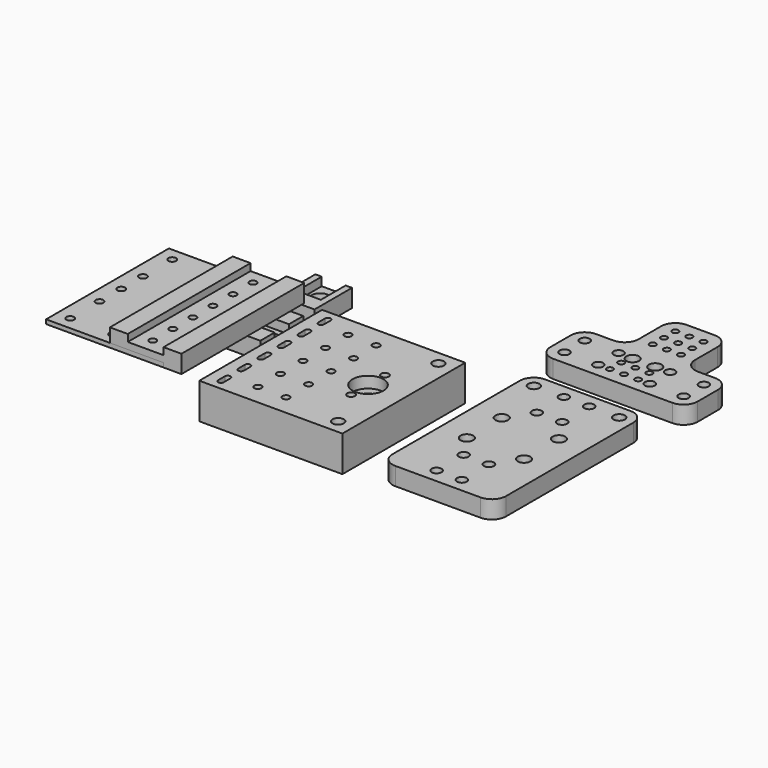
from build123d import *

# Parameters (mm, degrees)
F1_R      = 2.5
F2_DEPTH  = 12.7
F3_W      = 25.4
F3_H      = 109
F3_R      = 2.5
F4_DEPTH  = 5
F0_R      = 2.55
F0_R_2    = 4
F0_R_3    = 2.75
F0_R_4    = 11
F0_R_5    = 5.2625
F5_DEPTH  = 25.4
F6_DEPTH  = 8
F7_R      = 2.75
F8_DEPTH  = 3
F9_R      = 3.5
F9_R_2    = 4.5
F9_R_3    = 4
F9_R_4    = 2.25
F9_R_5    = 2.75
F10_DEPTH = 12.7
F11_DEPTH = 5
F12_R     = 3.5
F12_R_2   = 2.25
F12_R_3   = 4.5
F12_R_4   = 2.5
F12_R_5   = 2
F13_DEPTH = 12.7
F14_DEPTH = 5
F15_W     = 26
F15_H     = 12.7
F15_R     = 2.25
F16_DEPTH = 12.7
F17_DEPTH = 6.35
F18_W     = 17
F18_H     = 22
F18_R     = 6.25
F19_DEPTH = 12.7
F20_DEPTH = 6


# Not quite as in the source:
# - a length typed as a fraction of an inch, garbled in the dataset ("3 / 203.2 mm" for 3/8 in), is restored


with BuildPart() as f2:
    # F1 (on Top) → F2 (new body)
    with BuildSketch(Plane.XY):
        Polygon((-50.8, 0), (-25.4, 0), (-12.7, 0), (-12.7, 109), (-25.4, 109), (-50.8, 109), (-63.5, 109), (-63.5, 0), align=None)
        with Locations((-41.06, 10)):
            Circle(F1_R, mode=Mode.SUBTRACT)
        with Locations((-41.06, 27.8)):
            Circle(F1_R, mode=Mode.SUBTRACT)
        with Locations((-41.06, 45.6)):
            Circle(F1_R, mode=Mode.SUBTRACT)
        with Locations((-41.06, 63.4)):
            Circle(F1_R, mode=Mode.SUBTRACT)
        with Locations((-41.06, 81.2)):
            Circle(F1_R, mode=Mode.SUBTRACT)
        with Locations((-41.06, 99)):
            Circle(F1_R, mode=Mode.SUBTRACT)
    extrude(amount=F2_DEPTH)

    # F3 (on face) → F4 (cut)
    with BuildSketch(Plane.XY.offset(12.7)):
        with Locations((-38.1, 54.5)):
            Rectangle(F3_W, F3_H)
        with Locations((-41.06, 10)):
            Circle(F3_R, mode=Mode.SUBTRACT)
        with Locations((-41.06, 27.8)):
            Circle(F3_R, mode=Mode.SUBTRACT)
        with Locations((-41.06, 45.6)):
            Circle(F3_R, mode=Mode.SUBTRACT)
        with Locations((-41.06, 63.4)):
            Circle(F3_R, mode=Mode.SUBTRACT)
        with Locations((-41.06, 81.2)):
            Circle(F3_R, mode=Mode.SUBTRACT)
        with Locations((-41.06, 99)):
            Circle(F3_R, mode=Mode.SUBTRACT)
    extrude(amount=-F4_DEPTH, mode=Mode.SUBTRACT)


with BuildPart() as f5:
    # F0 (on Top) → F5 (new body)
    with BuildSketch(Plane.XY):
        Polygon((0, 109), (0, 0), (101.6, 0), (101.6, 102.8568819165), (101.6, 109), align=None)
        with BuildLine():
            ThreePointArc((7.74, 13), (9.74, 15), (11.74, 13))
            Line((11.74, 13), (11.74, 7))
            ThreePointArc((11.74, 7), (9.74, 5), (7.74, 7))
            Line((7.74, 7), (7.74, 13))
        make_face(mode=Mode.SUBTRACT)
        with Locations((30, 14.5)):
            Circle(F0_R, mode=Mode.SUBTRACT)
        with Locations((50, 14.5)):
            Circle(F0_R, mode=Mode.SUBTRACT)
        with BuildLine():
            ThreePointArc((7.74, 30.8), (9.74, 32.8), (11.74, 30.8))
            Line((11.74, 30.8), (11.74, 24.8))
            ThreePointArc((11.74, 24.8), (9.74, 22.8), (7.74, 24.8))
            Line((7.74, 24.8), (7.74, 30.8))
        make_face(mode=Mode.SUBTRACT)
        with BuildLine():
            ThreePointArc((7.74, 48.6), (9.74, 50.6), (11.74, 48.6))
            Line((11.74, 48.6), (11.74, 42.6))
            ThreePointArc((11.74, 42.6), (9.74, 40.6), (7.74, 42.6))
            Line((7.74, 42.6), (7.74, 48.6))
        make_face(mode=Mode.SUBTRACT)
        with Locations((30, 34.5)):
            Circle(F0_R, mode=Mode.SUBTRACT)
        with Locations((50, 34.5)):
            Circle(F0_R, mode=Mode.SUBTRACT)
        with Locations((90.6, 10)):
            Circle(F0_R_2, mode=Mode.SUBTRACT)
        with Locations((76.2, 39.5)):
            Circle(F0_R_3, mode=Mode.SUBTRACT)
        with BuildLine():
            ThreePointArc((7.74, 66.4), (9.74, 68.4), (11.74, 66.4))
            Line((11.74, 66.4), (11.74, 60.4))
            ThreePointArc((11.74, 60.4), (9.74, 58.4), (7.74, 60.4))
            Line((7.74, 60.4), (7.74, 66.4))
        make_face(mode=Mode.SUBTRACT)
        with BuildLine():
            ThreePointArc((7.74, 84.2), (9.74, 86.2), (11.74, 84.2))
            Line((11.74, 84.2), (11.74, 78.2))
            ThreePointArc((11.74, 78.2), (9.74, 76.2), (7.74, 78.2))
            Line((7.74, 78.2), (7.74, 84.2))
        make_face(mode=Mode.SUBTRACT)
        with Locations((30, 54.5)):
            Circle(F0_R, mode=Mode.SUBTRACT)
        with Locations((50, 54.5)):
            Circle(F0_R, mode=Mode.SUBTRACT)
        with Locations((30, 74.5)):
            Circle(F0_R, mode=Mode.SUBTRACT)
        with Locations((50, 74.5)):
            Circle(F0_R, mode=Mode.SUBTRACT)
        with BuildLine():
            ThreePointArc((7.74, 102), (9.74, 104), (11.74, 102))
            Line((11.74, 102), (11.74, 96))
            ThreePointArc((11.74, 96), (9.74, 94), (7.74, 96))
            Line((7.74, 96), (7.74, 102))
        make_face(mode=Mode.SUBTRACT)
        with Locations((30, 94.5)):
            Circle(F0_R, mode=Mode.SUBTRACT)
        with Locations((50, 94.5)):
            Circle(F0_R, mode=Mode.SUBTRACT)
        with Locations((76.2, 54.5)):
            Circle(F0_R_4, mode=Mode.SUBTRACT)
        with Locations((76.2, 69.5)):
            Circle(F0_R_3, mode=Mode.SUBTRACT)
        with Locations((90.6, 99)):
            Circle(F0_R_2, mode=Mode.SUBTRACT)
        with Locations((76.2, 54.5)):
            Circle(F0_R_4)
        with Locations((76.2, 54.5)):
            Circle(F0_R_5, mode=Mode.SUBTRACT)
    extrude(amount=-F5_DEPTH)

    # F0 (on Top) → F6 (cut)
    with BuildSketch(Plane.XY):
        with Locations((76.2, 54.5)):
            Circle(F0_R_4)
        with Locations((76.2, 54.5)):
            Circle(F0_R_5, mode=Mode.SUBTRACT)
    extrude(amount=-F6_DEPTH, mode=Mode.SUBTRACT)


with BuildPart() as f8:
    # F7 (on face) → F8 (new body)
    with BuildSketch(Plane.XY):
        Polygon((-25.4, 0), (-25.4, 109), (-58.8, 109), (-83.8, 109), (-108.8, 109), (-108.8, 0), align=None)
        with Locations((-99.05, 9.25)):
            Circle(F7_R, mode=Mode.SUBTRACT)
        with Locations((-68.55, 9.25)):
            Circle(F7_R, mode=Mode.SUBTRACT)
        with Locations((-35.14, 10)):
            Circle(F7_R, mode=Mode.SUBTRACT)
        with Locations((-99.05, 35.25)):
            Circle(F7_R, mode=Mode.SUBTRACT)
        with Locations((-68.55, 35.25)):
            Circle(F7_R, mode=Mode.SUBTRACT)
        with Locations((-35.14, 27.8)):
            Circle(F7_R, mode=Mode.SUBTRACT)
        with Locations((-35.14, 45.6)):
            Circle(F7_R, mode=Mode.SUBTRACT)
        with Locations((-99.05, 54.5)):
            Circle(F7_R, mode=Mode.SUBTRACT)
        with Locations((-68.55, 54.5)):
            Circle(F7_R, mode=Mode.SUBTRACT)
        with Locations((-99.05, 73.75)):
            Circle(F7_R, mode=Mode.SUBTRACT)
        with Locations((-68.55, 73.75)):
            Circle(F7_R, mode=Mode.SUBTRACT)
        with Locations((-35.14, 63.4)):
            Circle(F7_R, mode=Mode.SUBTRACT)
        with Locations((-35.14, 81.2)):
            Circle(F7_R, mode=Mode.SUBTRACT)
        with Locations((-99.05, 99.75)):
            Circle(F7_R, mode=Mode.SUBTRACT)
        with Locations((-68.55, 99.75)):
            Circle(F7_R, mode=Mode.SUBTRACT)
        with Locations((-35.14, 99)):
            Circle(F7_R, mode=Mode.SUBTRACT)
    extrude(amount=F8_DEPTH)


with BuildPart() as f10:
    # F9 (on face) → F10 (new body)
    with BuildSketch(Plane.XY):
        with BuildLine():
            ThreePointArc((138.7726175785, -2), (141.7015497666, -9.0710678119), (148.7726175785, -12))
            Line((148.7726175785, -12), (209.3726175785, -12))
            ThreePointArc((209.3726175785, -12), (216.4436853904, -9.0710678119), (219.3726175785, -2))
            Line((219.3726175785, -2), (219.3726175785, 111))
            ThreePointArc((219.3726175785, 111), (216.4436853904, 118.0710678119), (209.3726175785, 121))
            Line((209.3726175785, 121), (148.7726175785, 121))
            ThreePointArc((148.7726175785, 121), (141.7015497666, 118.0710678119), (138.7726175785, 111))
            Line((138.7726175785, 111), (138.7726175785, -2))
        make_face()
        with Locations((170.0726175785, -2)):
            Circle(F9_R, mode=Mode.SUBTRACT)
        with Locations((188.0726175785, -2)):
            Circle(F9_R, mode=Mode.SUBTRACT)
        with Locations((158.7726175785, 39)):
            Circle(F9_R_2, mode=Mode.SUBTRACT)
        with Locations((170.0726175785, 22)):
            Circle(F9_R, mode=Mode.SUBTRACT)
        with Locations((188.0726175785, 22)):
            Circle(F9_R, mode=Mode.SUBTRACT)
        with Locations((199.3726175785, 39)):
            Circle(F9_R_2, mode=Mode.SUBTRACT)
        with Locations((158.7726175785, 70)):
            Circle(F9_R_2, mode=Mode.SUBTRACT)
        with Locations((199.3726175785, 70)):
            Circle(F9_R_2, mode=Mode.SUBTRACT)
        with Locations((170.0726175785, 87)):
            Circle(F9_R, mode=Mode.SUBTRACT)
        with Locations((188.0726175785, 87)):
            Circle(F9_R, mode=Mode.SUBTRACT)
        with Locations((148.7726175785, 111)):
            Circle(F9_R_3, mode=Mode.SUBTRACT)
        with Locations((170.0726175785, 111)):
            Circle(F9_R, mode=Mode.SUBTRACT)
        with Locations((188.0726175785, 111)):
            Circle(F9_R, mode=Mode.SUBTRACT)
        with Locations((209.3726175785, 111)):
            Circle(F9_R_3, mode=Mode.SUBTRACT)
        with Locations((170.0726175785, 111)):
            Circle(F9_R)
        with Locations((170.0726175785, 111)):
            Circle(F9_R_4, mode=Mode.SUBTRACT)
        with Locations((170.0726175785, 87)):
            Circle(F9_R)
        with Locations((170.0726175785, 87)):
            Circle(F9_R_4, mode=Mode.SUBTRACT)
        with Locations((188.0726175785, 87)):
            Circle(F9_R)
        with Locations((188.0726175785, 87)):
            Circle(F9_R_4, mode=Mode.SUBTRACT)
        with Locations((188.0726175785, 111)):
            Circle(F9_R)
        with Locations((188.0726175785, 111)):
            Circle(F9_R_4, mode=Mode.SUBTRACT)
        with Locations((158.7726175785, 70)):
            Circle(F9_R_2)
        with Locations((158.7726175785, 70)):
            Circle(F9_R_5, mode=Mode.SUBTRACT)
        with Locations((158.7726175785, 39)):
            Circle(F9_R_2)
        with Locations((158.7726175785, 39)):
            Circle(F9_R_5, mode=Mode.SUBTRACT)
        with Locations((199.3726175785, 39)):
            Circle(F9_R_2)
        with Locations((199.3726175785, 39)):
            Circle(F9_R_5, mode=Mode.SUBTRACT)
        with Locations((199.3726175785, 70)):
            Circle(F9_R_2)
        with Locations((199.3726175785, 70)):
            Circle(F9_R_5, mode=Mode.SUBTRACT)
        with Locations((170.0726175785, 22)):
            Circle(F9_R)
        with Locations((170.0726175785, 22)):
            Circle(F9_R_4, mode=Mode.SUBTRACT)
        with Locations((170.0726175785, -2)):
            Circle(F9_R)
        with Locations((170.0726175785, -2)):
            Circle(F9_R_4, mode=Mode.SUBTRACT)
        with Locations((188.0726175785, -2)):
            Circle(F9_R)
        with Locations((188.0726175785, -2)):
            Circle(F9_R_4, mode=Mode.SUBTRACT)
        with Locations((188.0726175785, 22)):
            Circle(F9_R)
        with Locations((188.0726175785, 22)):
            Circle(F9_R_4, mode=Mode.SUBTRACT)
    extrude(amount=-F10_DEPTH)

    # F9 (on face) → F11 (cut)
    with BuildSketch(Plane.XY):
        with Locations((158.7726175785, 70)):
            Circle(F9_R_2)
        with Locations((158.7726175785, 70)):
            Circle(F9_R_5, mode=Mode.SUBTRACT)
        with Locations((170.0726175785, 111)):
            Circle(F9_R)
        with Locations((170.0726175785, 111)):
            Circle(F9_R_4, mode=Mode.SUBTRACT)
        with Locations((188.0726175785, 111)):
            Circle(F9_R)
        with Locations((188.0726175785, 111)):
            Circle(F9_R_4, mode=Mode.SUBTRACT)
        with Locations((188.0726175785, 87)):
            Circle(F9_R)
        with Locations((188.0726175785, 87)):
            Circle(F9_R_4, mode=Mode.SUBTRACT)
        with Locations((170.0726175785, 87)):
            Circle(F9_R)
        with Locations((170.0726175785, 87)):
            Circle(F9_R_4, mode=Mode.SUBTRACT)
        with Locations((199.3726175785, 70)):
            Circle(F9_R_2)
        with Locations((199.3726175785, 70)):
            Circle(F9_R_5, mode=Mode.SUBTRACT)
        with Locations((158.7726175785, 39)):
            Circle(F9_R_2)
        with Locations((158.7726175785, 39)):
            Circle(F9_R_5, mode=Mode.SUBTRACT)
        with Locations((199.3726175785, 39)):
            Circle(F9_R_2)
        with Locations((199.3726175785, 39)):
            Circle(F9_R_5, mode=Mode.SUBTRACT)
        with Locations((188.0726175785, 22)):
            Circle(F9_R)
        with Locations((188.0726175785, 22)):
            Circle(F9_R_4, mode=Mode.SUBTRACT)
        with Locations((170.0726175785, 22)):
            Circle(F9_R)
        with Locations((170.0726175785, 22)):
            Circle(F9_R_4, mode=Mode.SUBTRACT)
        with Locations((188.0726175785, -2)):
            Circle(F9_R)
        with Locations((188.0726175785, -2)):
            Circle(F9_R_4, mode=Mode.SUBTRACT)
        with Locations((170.0726175785, -2)):
            Circle(F9_R)
        with Locations((170.0726175785, -2)):
            Circle(F9_R_4, mode=Mode.SUBTRACT)
    extrude(amount=-F11_DEPTH, mode=Mode.SUBTRACT)


with BuildPart() as f13:
    # F12 (on face) → F13 (new body)
    with BuildSketch(Plane.XY):
        with BuildLine():
            Line((136.7726175785, 143.165299654), (221.3726175785, 143.165299654))
            ThreePointArc((221.3726175785, 143.165299654), (228.4436853904, 146.0942318421), (231.3726175785, 153.165299654))
            Line((231.3726175785, 153.165299654), (231.3726175785, 171.165299654))
            ThreePointArc((231.3726175785, 171.165299654), (228.4436853904, 178.2363674659), (221.3726175785, 181.165299654))
            Line((221.3726175785, 181.165299654), (209.0726175785, 181.165299654))
            ThreePointArc((209.0726175785, 181.165299654), (202.0015497666, 184.0942318421), (199.0726175785, 191.165299654))
            Line((199.0726175785, 191.165299654), (199.0726175785, 211.165299654))
            ThreePointArc((199.0726175785, 211.165299654), (196.1436853904, 218.2363674659), (189.0726175785, 221.165299654))
            Line((189.0726175785, 221.165299654), (169.0726175785, 221.165299654))
            ThreePointArc((169.0726175785, 221.165299654), (162.0015497666, 218.2363674659), (159.0726175785, 211.165299654))
            Line((159.0726175785, 211.165299654), (159.0726175785, 191.165299654))
            ThreePointArc((159.0726175785, 191.165299654), (156.1436853904, 184.0942318421), (149.0726175785, 181.165299654))
            Line((149.0726175785, 181.165299654), (136.7726175785, 181.165299654))
            ThreePointArc((136.7726175785, 181.165299654), (129.7015497666, 178.2363674659), (126.7726175785, 171.165299654))
            Line((126.7726175785, 171.165299654), (126.7726175785, 153.165299654))
            ThreePointArc((126.7726175785, 153.165299654), (129.7015497666, 146.0942318421), (136.7726175785, 143.165299654))
        make_face()
        with Locations((136.7726175785, 153.165299654)):
            Circle(F12_R, mode=Mode.SUBTRACT)
        with Locations((160.7726175785, 153.165299654)):
            Circle(F12_R, mode=Mode.SUBTRACT)
        with Locations((169.0726175785, 153.165299654)):
            Circle(F12_R_2, mode=Mode.SUBTRACT)
        with Locations((179.0726175785, 153.165299654)):
            Circle(F12_R_2, mode=Mode.SUBTRACT)
        with Locations((136.7726175785, 171.165299654)):
            Circle(F12_R, mode=Mode.SUBTRACT)
        with Locations((160.7726175785, 171.165299654)):
            Circle(F12_R, mode=Mode.SUBTRACT)
        with Locations((169.0726175785, 163.165299654)):
            Circle(F12_R_2, mode=Mode.SUBTRACT)
        with Locations((171.0726175785, 170.815299654)):
            Circle(F12_R_3, mode=Mode.SUBTRACT)
        with Locations((179.0726175785, 163.165299654)):
            Circle(F12_R_2, mode=Mode.SUBTRACT)
        with Locations((169.0726175785, 191.165299654)):
            Circle(F12_R_2, mode=Mode.SUBTRACT)
        with BuildLine():
            ThreePointArc((181.3226175785, 191.165299654), (179.0726175785, 188.915299654), (176.8226175785, 191.165299654))
            ThreePointArc((176.8226175785, 191.165299654), (179.0726175785, 193.415299654), (181.3226175785, 191.165299654))
        make_face(mode=Mode.SUBTRACT)
        with Locations((169.0726175785, 201.165299654)):
            Circle(F12_R_2, mode=Mode.SUBTRACT)
        with Locations((179.0726175785, 201.165299654)):
            Circle(F12_R_2, mode=Mode.SUBTRACT)
        with Locations((169.0726175785, 211.165299654)):
            Circle(F12_R_2, mode=Mode.SUBTRACT)
        with Locations((179.0726175785, 211.165299654)):
            Circle(F12_R_2, mode=Mode.SUBTRACT)
        with Locations((189.0726175785, 153.165299654)):
            Circle(F12_R_2, mode=Mode.SUBTRACT)
        with Locations((197.3726175785, 153.165299654)):
            Circle(F12_R, mode=Mode.SUBTRACT)
        with Locations((221.3726175785, 153.165299654)):
            Circle(F12_R, mode=Mode.SUBTRACT)
        with Locations((189.0726175785, 163.165299654)):
            Circle(F12_R_2, mode=Mode.SUBTRACT)
        with Locations((187.0726175785, 170.815299654)):
            Circle(F12_R_3, mode=Mode.SUBTRACT)
        with BuildLine():
            ThreePointArc((191.3226175785, 191.165299654), (189.0726175785, 188.915299654), (186.8226175785, 191.165299654))
            ThreePointArc((186.8226175785, 191.165299654), (189.0726175785, 193.415299654), (191.3226175785, 191.165299654))
        make_face(mode=Mode.SUBTRACT)
        with Locations((197.3726175785, 171.165299654)):
            Circle(F12_R, mode=Mode.SUBTRACT)
        with Locations((189.0726175785, 201.165299654)):
            Circle(F12_R_2, mode=Mode.SUBTRACT)
        with Locations((189.0726175785, 211.165299654)):
            Circle(F12_R_2, mode=Mode.SUBTRACT)
        with Locations((221.3726175785, 171.165299654)):
            Circle(F12_R, mode=Mode.SUBTRACT)
        with Locations((171.0726175785, 170.815299654)):
            Circle(F12_R_3)
        with Locations((171.0726175785, 170.815299654)):
            Circle(F12_R_4, mode=Mode.SUBTRACT)
        with Locations((187.0726175785, 170.815299654)):
            Circle(F12_R_3)
        with Locations((187.0726175785, 170.815299654)):
            Circle(F12_R_4, mode=Mode.SUBTRACT)
        with Locations((136.7726175785, 171.165299654)):
            Circle(F12_R)
        with Locations((136.7726175785, 171.165299654)):
            Circle(F12_R_5, mode=Mode.SUBTRACT)
        with Locations((136.7726175785, 153.165299654)):
            Circle(F12_R)
        with Locations((136.7726175785, 153.165299654)):
            Circle(F12_R_5, mode=Mode.SUBTRACT)
        with Locations((160.7726175785, 171.165299654)):
            Circle(F12_R)
        with Locations((160.7726175785, 171.165299654)):
            Circle(F12_R_5, mode=Mode.SUBTRACT)
        with Locations((160.7726175785, 153.165299654)):
            Circle(F12_R)
        with Locations((160.7726175785, 153.165299654)):
            Circle(F12_R_5, mode=Mode.SUBTRACT)
        with Locations((197.3726175785, 171.165299654)):
            Circle(F12_R)
        with Locations((197.3726175785, 171.165299654)):
            Circle(F12_R_5, mode=Mode.SUBTRACT)
        with Locations((197.3726175785, 153.165299654)):
            Circle(F12_R)
        with Locations((197.3726175785, 153.165299654)):
            Circle(F12_R_5, mode=Mode.SUBTRACT)
        with Locations((221.3726175785, 171.165299654)):
            Circle(F12_R)
        with Locations((221.3726175785, 171.165299654)):
            Circle(F12_R_5, mode=Mode.SUBTRACT)
        with Locations((221.3726175785, 153.165299654)):
            Circle(F12_R)
        with Locations((221.3726175785, 153.165299654)):
            Circle(F12_R_5, mode=Mode.SUBTRACT)
    extrude(amount=-F13_DEPTH)

    # F12 (on face) → F14 (cut)
    with BuildSketch(Plane.XY):
        with Locations((160.7726175785, 171.165299654)):
            Circle(F12_R)
        with Locations((160.7726175785, 171.165299654)):
            Circle(F12_R_5, mode=Mode.SUBTRACT)
        with Locations((136.7726175785, 171.165299654)):
            Circle(F12_R)
        with Locations((136.7726175785, 171.165299654)):
            Circle(F12_R_5, mode=Mode.SUBTRACT)
        with Locations((136.7726175785, 153.165299654)):
            Circle(F12_R)
        with Locations((136.7726175785, 153.165299654)):
            Circle(F12_R_5, mode=Mode.SUBTRACT)
        with Locations((160.7726175785, 153.165299654)):
            Circle(F12_R)
        with Locations((160.7726175785, 153.165299654)):
            Circle(F12_R_5, mode=Mode.SUBTRACT)
        with Locations((171.0726175785, 170.815299654)):
            Circle(F12_R_3)
        with Locations((171.0726175785, 170.815299654)):
            Circle(F12_R_4, mode=Mode.SUBTRACT)
        with Locations((187.0726175785, 170.815299654)):
            Circle(F12_R_3)
        with Locations((187.0726175785, 170.815299654)):
            Circle(F12_R_4, mode=Mode.SUBTRACT)
        with Locations((197.3726175785, 171.165299654)):
            Circle(F12_R)
        with Locations((197.3726175785, 171.165299654)):
            Circle(F12_R_5, mode=Mode.SUBTRACT)
        with Locations((221.3726175785, 171.165299654)):
            Circle(F12_R)
        with Locations((221.3726175785, 171.165299654)):
            Circle(F12_R_5, mode=Mode.SUBTRACT)
        with Locations((221.3726175785, 153.165299654)):
            Circle(F12_R)
        with Locations((221.3726175785, 153.165299654)):
            Circle(F12_R_5, mode=Mode.SUBTRACT)
        with Locations((197.3726175785, 153.165299654)):
            Circle(F12_R)
        with Locations((197.3726175785, 153.165299654)):
            Circle(F12_R_5, mode=Mode.SUBTRACT)
    extrude(amount=-F14_DEPTH, mode=Mode.SUBTRACT)


with BuildPart() as f16:
    # F15 (on Top) → F16 (new body)
    with BuildSketch(Plane.XY):
        with Locations((-16.5686666848, 90.3771459834)):
            Rectangle(F15_W, F15_H)
        with Locations((-16.5686666848, 77.6771459834)):
            Rectangle(F15_W, F15_H)
        with Locations((-24.5686666848, 77.6771459834)):
            Circle(F15_R, mode=Mode.SUBTRACT)
        with Locations((-8.5686666848, 77.6771459834)):
            Circle(F15_R, mode=Mode.SUBTRACT)
        with Locations((-16.5686666848, 64.9771459834)):
            Rectangle(F15_W, F15_H)
    extrude(amount=-F16_DEPTH)

    # F15 (on Top) → F17 (cut)
    with BuildSketch(Plane.XY):
        with Locations((-16.5686666848, 77.6771459834)):
            Rectangle(F15_W, F15_H)
        with Locations((-24.5686666848, 77.6771459834)):
            Circle(F15_R, mode=Mode.SUBTRACT)
        with Locations((-8.5686666848, 77.6771459834)):
            Circle(F15_R, mode=Mode.SUBTRACT)
    extrude(amount=-F17_DEPTH, mode=Mode.SUBTRACT)


with BuildPart() as f19:
    # F18 (on Top) → F19 (new body)
    with BuildSketch(Plane.XY):
        with Locations((-16.5686666848, 128.9771459834)):
            Rectangle(F18_W, F18_H)
        with Locations((-16.5686666848, 127.9771459834)):
            Circle(F18_R, mode=Mode.SUBTRACT)
        Polygon((-29.5686666848, 139.9771459834), (-29.5686666848, 106.7271459834), (-3.5686666848, 106.7271459834), (-3.5686666848, 139.9771459834), (-8.0686666848, 139.9771459834), (-8.0686666848, 117.9771459834), (-25.0686666848, 117.9771459834), (-25.0686666848, 139.9771459834), align=None)
    extrude(amount=-F19_DEPTH)

    # F18 (on Top) → F20 (cut)
    with BuildSketch(Plane.XY):
        with Locations((-16.5686666848, 128.9771459834)):
            Rectangle(F18_W, F18_H)
        with Locations((-16.5686666848, 127.9771459834)):
            Circle(F18_R, mode=Mode.SUBTRACT)
    extrude(amount=-F20_DEPTH, mode=Mode.SUBTRACT)


solid = Compound([f2.part, f5.part, f8.part, f10.part, f13.part, f16.part, f19.part])
